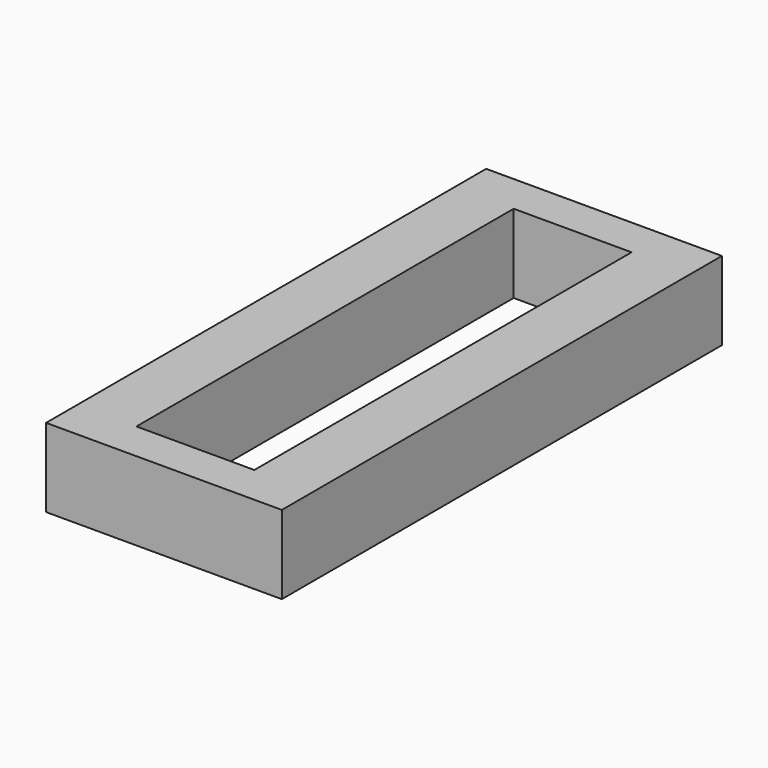
from build123d import *

# Parameters (mm, degrees)
F0_W     = 76.2
F0_H     = 25.4
F1_DEPTH = 88.9
F2_W     = 38.1
F2_H     = 152.4
F3_DEPTH = 38.1


# Not quite as in the source:
# - a feature of the source that left no trace in its solid (it failed there, or was rolled back) is left out


with BuildPart() as f1:
    # F0 (on Front) → F1 (new body, symmetric)
    with BuildSketch(Plane.XZ):
        Rectangle(F0_W, F0_H)
    extrude(amount=F1_DEPTH, both=True)

    # F2 (on face) → F3 (cut)
    with BuildSketch(Plane.XY.offset(12.7)):
        Rectangle(F2_W, F2_H)
    extrude(amount=-F3_DEPTH, mode=Mode.SUBTRACT)


solid = f1.part
